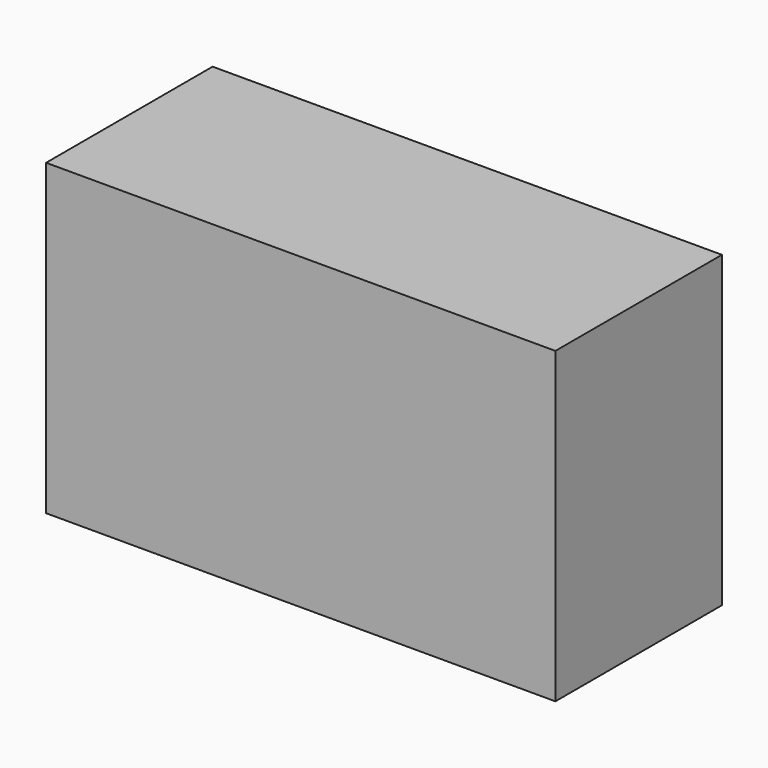
from build123d import *

# Parameters (mm, degrees)
F0_W     = 31.6992029548
F0_H     = 19.2023999989
F0_R     = 4.5234834091
F0_R_2   = 4.8791801503
F1_DEPTH = 12.954


# Not quite as in the source:
# - the program builds the solid bodies; features that only make, move or delete a surface that nothing else refers to are left out


with BuildPart() as f1:
    # F0 (on Front) → F1 (new body)
    with BuildSketch(Plane.XZ):
        Rectangle(F0_W, F0_H)
        with Locations((-9.1440007091, 0)):
            Circle(F0_R, mode=Mode.SUBTRACT)
        with Locations((8.8392002508, 0)):
            Circle(F0_R_2, mode=Mode.SUBTRACT)
        with Locations((-9.1440007091, 0)):
            Circle(F0_R)
        with Locations((8.8392002508, 0)):
            Circle(F0_R_2)
    extrude(amount=F1_DEPTH)


solid = f1.part
